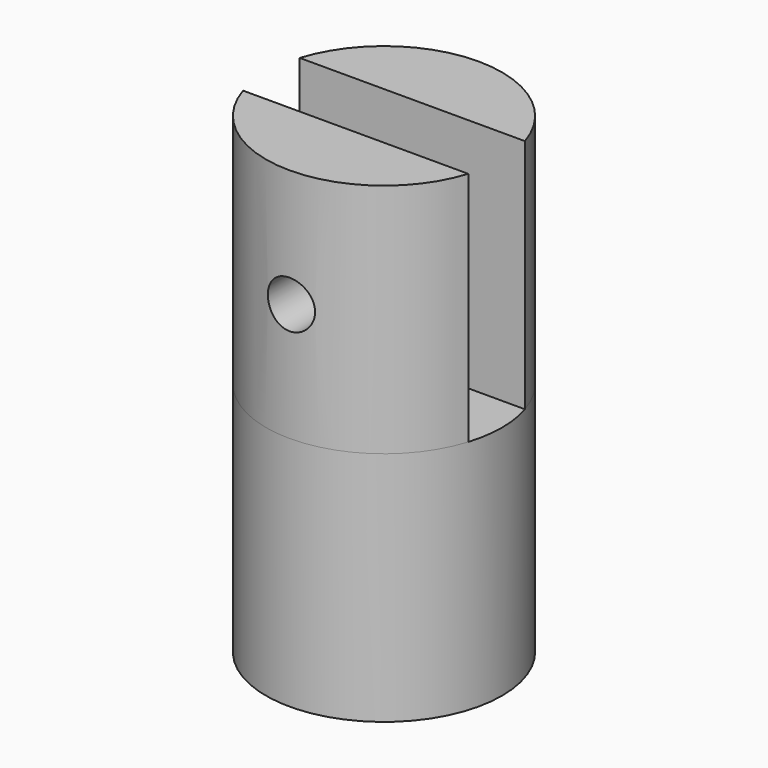
from build123d import *

# Parameters (mm, degrees)
F0_R     = 25
F1_DEPTH = 50
F3_DEPTH = 50
F5_R     = 5
F6_DEPTH = 25


# Not quite as in the source:
# - after a boolean that leaves OpenCascade's solid faulty, fix() repairs it


with BuildPart() as f1:
    # F0 (on Top) → F1 (new body)
    with BuildSketch(Plane.XY):
        Circle(F0_R)
    extrude(amount=F1_DEPTH)

    # F2 (on face) → F3 (join)
    with BuildSketch(Plane.XY.offset(50)):
        with BuildLine():
            Line((23.8484800354, -7.5), (-23.8484800354, -7.5))
            ThreePointArc((-23.8484800354, -7.5), (0, -25), (23.8484800354, -7.5))
        make_face()
    extrude(amount=F3_DEPTH)

    # F4: F1 across plane


with BuildPart() as f1_1:
    add(f1.part)
    add(f1.part.mirror(Plane.XZ))

    add(f1_1.part.fix(), mode=Mode.REPLACE)

    # F5 (on Front) → F6 (cut, symmetric)
    with BuildSketch(Plane.XZ):
        with Locations((0, 75)):
            Circle(F5_R)
    extrude(amount=F6_DEPTH, both=True, mode=Mode.SUBTRACT)


solid = f1_1.part
